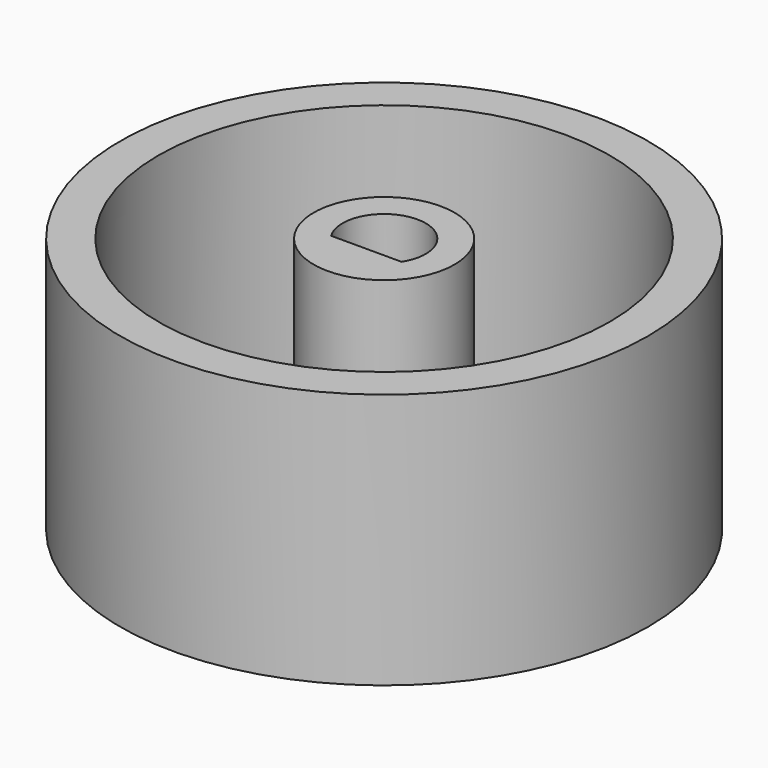
from build123d import *

# Parameters (mm, degrees)
F0_R     = 10.4775
F1_DEPTH = 1.27
F2_R     = 10.4775
F2_R_2   = 8.9535
F2_R_3   = 2.794
F3_DEPTH = 8.89


# Not quite as in the source:
# - the program builds the solid bodies; features that only make, move or delete a surface that nothing else refers to are left out


with BuildPart() as f1:
    # F0 (on Top) → F1 (new body)
    with BuildSketch(Plane.XY):
        Circle(F0_R)
    extrude(amount=F1_DEPTH)

    # F2 (on face) → F3 (join)
    with BuildSketch(Plane.XY.offset(1.27)):
        Circle(F2_R)
        Circle(F2_R_2, mode=Mode.SUBTRACT)
        Circle(F2_R_3)
        with BuildLine():
            ThreePointArc((-1.397, -0.8798818102), (0, 1.651), (1.397, -0.8798818102))
            Line((1.397, -0.8798818102), (-1.397, -0.8798818102))
        make_face(mode=Mode.SUBTRACT)
    extrude(amount=F3_DEPTH)


solid = f1.part
